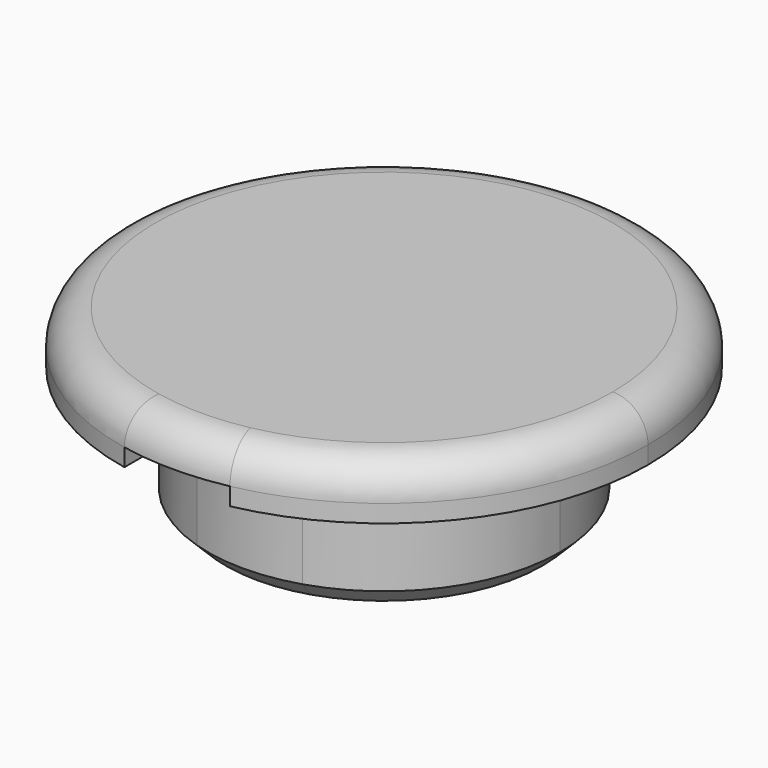
from build123d import *
from build123d import SkipClean  # not in build123d's __all__

# Parameters (mm, degrees)
F0_R     = 8
F1_DEPTH = 3
F2_DEPTH = 7
F3_R     = 2
F4_SIZE  = 1
F5_DEPTH = 1


with BuildPart() as f1:
    # F0 (on Top) → F1 (new body)
    with BuildSketch(Plane.XY):
        with BuildLine():
            ThreePointArc((-3, -9.5393920142), (-5.9160797831, 8.0622577483), (10, 0))
            ThreePointArc((10, 0), (8.0622577483, -5.9160797831), (3, -9.5393920142))
            Line((3, -9.5393920142), (3, -14.6969384567))
            ThreePointArc((3, -14.6969384567), (11.6189500386, -9.4868329805), (15, 0))
            ThreePointArc((15, 0), (-9.4868329805, 11.6189500386), (-3, -14.6969384567))
            Line((-3, -14.6969384567), (-3, -9.5393920142))
        make_face()
        with BuildLine():
            ThreePointArc((3, -9.5393920142), (0, -10), (-3, -9.5393920142))
            Line((-3, -9.5393920142), (-3, -14.6969384567))
            ThreePointArc((-3, -14.6969384567), (0, -15), (3, -14.6969384567))
            Line((3, -14.6969384567), (3, -9.5393920142))
        make_face()
        with BuildLine():
            ThreePointArc((3, -9.5393920142), (8.0622577483, -5.9160797831), (10, 0))
            ThreePointArc((10, 0), (-5.9160797831, 8.0622577483), (-3, -9.5393920142))
            ThreePointArc((-3, -9.5393920142), (0, -10), (3, -9.5393920142))
        make_face()
        Circle(F0_R, mode=Mode.SUBTRACT)
        Circle(F0_R)
    extrude(amount=F1_DEPTH)

    # F0 (on Top) → F2 (join)
    with BuildSketch(Plane.XY):
        with BuildLine():
            ThreePointArc((3, -9.5393920142), (8.0622577483, -5.9160797831), (10, 0))
            ThreePointArc((10, 0), (-5.9160797831, 8.0622577483), (-3, -9.5393920142))
            ThreePointArc((-3, -9.5393920142), (0, -10), (3, -9.5393920142))
        make_face()
        Circle(F0_R, mode=Mode.SUBTRACT)
    extrude(amount=-F2_DEPTH)

    # F3
    f3_edges = [f1.edges().sort_by_distance(p)[0] for p in [
        (-15, 0, 3),
    ]]
    fillet(f3_edges, radius=F3_R)

    # F4
    f4_edges = [f1.edges().sort_by_distance(p)[0] for p in [
        (3, 9.539392, -7),
    ]]
    chamfer(f4_edges, length=F4_SIZE)

    # F0 (on Top) → F5 (cut)
    with BuildSketch(Plane.XY):
        with BuildLine():
            ThreePointArc((3, -9.5393920142), (0, -10), (-3, -9.5393920142))
            Line((-3, -9.5393920142), (-3, -14.6969384567))
            ThreePointArc((-3, -14.6969384567), (0, -15), (3, -14.6969384567))
            Line((3, -14.6969384567), (3, -9.5393920142))
        make_face()
    with SkipClean():  # cleaning this boolean's faces spoils the solid; the shape is the same uncleaned
        extrude(amount=F5_DEPTH, mode=Mode.SUBTRACT)


solid = f1.part
